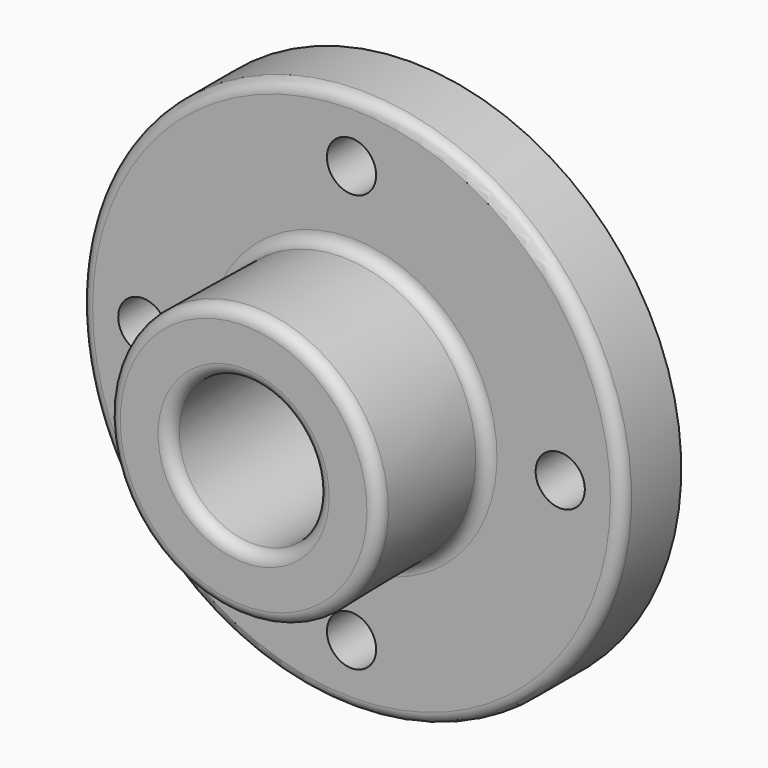
from build123d import *

# Parameters (mm, degrees)
F2_R            = 19.0246
F3_DEPTH        = 53.849
F4_R            = 6.35
F5_DEPTH        = 53.849
F5_COPIES_COUNT = 4
F6_R            = 3.048


# Not quite as in the source:
# - a pattern or mirror of a feature is missing from the dataset's text; its kind, count and spacing are read off the source's solid


with BuildPart() as f1:
    # F0 (on Right) → F1 (revolve)
    with BuildSketch(Plane.YZ):
        Polygon((34.798, 34.4624179433), (0, 34.925), (0, 0), (53.848, 0), (53.848, 69.85), (34.798, 69.85), align=None)
    revolve(axis=Axis((0, 26.924, 0), (0, 1, 0)))

    # F2 (on Front) → F3 (cut, through all)
    with BuildSketch(Plane.XZ):
        Circle(F2_R)
    extrude(amount=-F3_DEPTH, mode=Mode.SUBTRACT)

    # F4 (on Front) → F5 (cut, through all)
    with BuildSketch(Plane.XZ):
        with Locations((0, 53.848)):
            Circle(F4_R)
    f5 = extrude(amount=-F5_DEPTH, mode=Mode.SUBTRACT)

    # F5_copies: F5 ×4 about axis
    f5_copies_axis = Axis((0, 0, 0), (0, 1, 0))
    for i in range(1, F5_COPIES_COUNT):
        add(f5.rotate(f5_copies_axis, i * 360 / F5_COPIES_COUNT), mode=Mode.SUBTRACT)

    # F6
    f6_edges = [f1.edges().sort_by_distance(p)[0] for p in [
        (0, 0, -34.925),
        (-19.0246, 0, 0),
        (0, 34.798, -69.85),
        (0, 34.798, -34.462418),
    ]]
    fillet(f6_edges, radius=F6_R)


solid = f1.part
